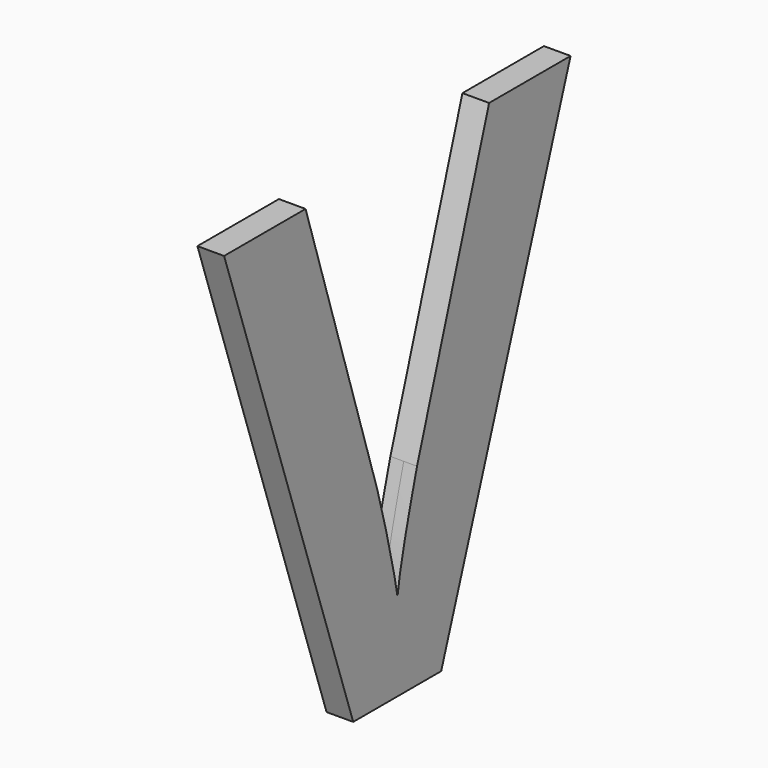
from build123d import *

# Parameters (mm, degrees)
F0_TEXT_SIZE = 635
F1_DEPTH     = 12.7


# Not quite as in the source:
# - Text() gives the source's letters only with a copy of the font that has no kerning and outlines rounded to 1/6400 em; it was checked with that copy


with BuildPart() as f1:
    # F0 (on Right) → F1 (new body, symmetric)
    with BuildSketch(Plane.YZ):
        with Locations((-412.65078125, 0)):
            Text('V', F0_TEXT_SIZE, font='Open Sans', font_style=FontStyle.BOLD, text_align=(TextAlign.LEFT, TextAlign.BOTTOM))
    extrude(amount=F1_DEPTH, both=True)


solid = f1.part
